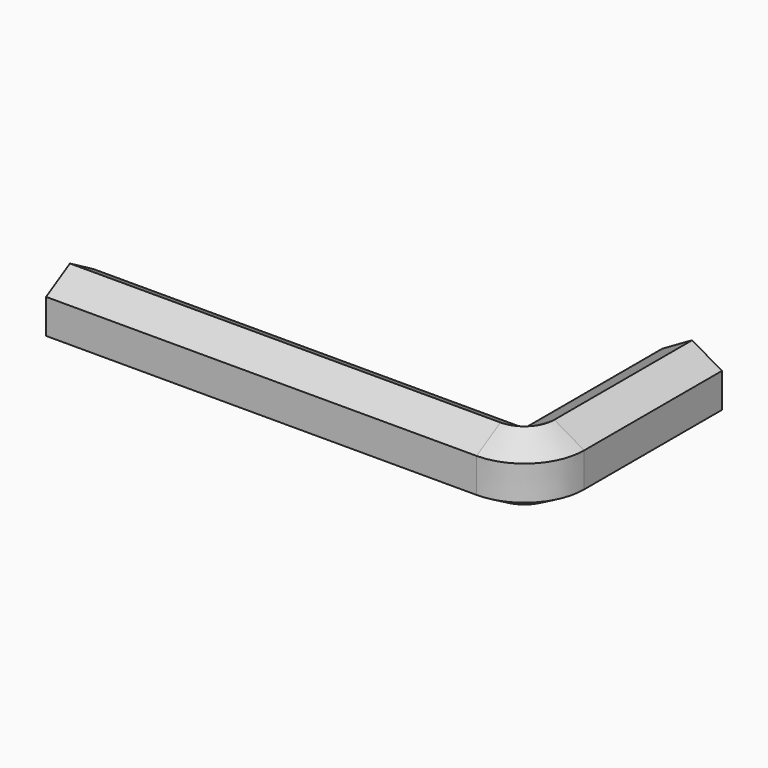
from build123d import *

# Parameters (mm, degrees)
F1_ANGLE = 90
F2_DEPTH = 60
F4_DEPTH = 150


with BuildPart() as f1:
    # F0 (on Front) → F1 (revolve)
    with BuildSketch(Plane.XZ):
        Polygon((-0.0259582262, -11.9999719237), (10.3793014176, -6.0224664452), (10.4052596438, 5.9775054785), (0.0259582262, 11.9999719237), (-10.3793014176, 6.0224664452), (-10.4052596438, -5.9775054785), align=None)
    revolve(axis=Axis((-10.4052596438, 0, 8.529782465), (0, 0, -1)), revolution_arc=F1_ANGLE)

    # F0 (on Front) → F2 (join)
    with BuildSketch(Plane.XZ):
        Polygon((-0.0259582262, -11.9999719237), (10.3793014176, -6.0224664452), (10.4052596438, 5.9775054785), (0.0259582262, 11.9999719237), (-10.3793014176, 6.0224664452), (-10.4052596438, -5.9775054785), align=None)
    extrude(amount=-F2_DEPTH)

    # F3 (on face) → F4 (join)
    with BuildSketch(Plane(origin=(-10.4052596438, 0, 0), x_dir=(0, -1, 0), z_dir=(-1, 0, 0))):
        Polygon((0, -5.9775054785), (10.3793014176, -11.9999719237), (20.7845610613, -6.0224664452), (20.8105192875, 5.9775054785), (10.43121787, 11.9999719237), (0.0259582262, 6.0224664452), align=None)
    extrude(amount=F4_DEPTH)


solid = f1.part
